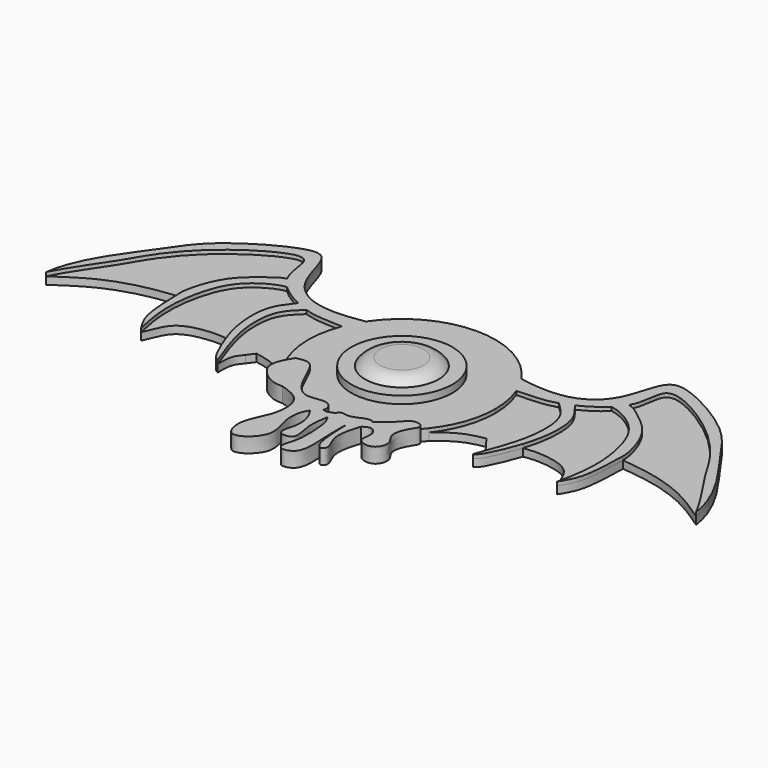
from build123d import *

# Parameters (mm, degrees)
F1_DEPTH  = 3
F2_R      = 13.5064277213
F3_DEPTH  = 5
F4_R      = 9.8042212389
F5_DEPTH  = 7
F7_DEPTH  = 2
F8_DEPTH  = 3
F10_DEPTH = 4


# Not quite as in the source:
# - a fillet or chamfer that OpenCascade refuses, or shapes differently, is made with other operations: its cross-section is extruded or revolved along the edge and cut away or added


with BuildPart() as f1:
    # F0 (on Top) → F1 (new body)
    with BuildSketch(Plane.XY):
        with BuildLine():
            ThreePointArc((-19.6218875172, -15.4913372651), (0, -25), (19.6218875172, -15.4913372651))
            add(Edge.make_bspline(
                [(20.7636337812, 13.92377507), (18.884492427, 12.8973675107), (13.2694896297, 9.830391573), (17.0839746859, -5.3747888898), (19.6218875172, -15.4913372651)],
                knots=[0, 0, 0, 0, 0.3346643665, 1, 1, 1, 1], degree=3))
            ThreePointArc((20.7636337812, 13.92377507), (0, 25), (-20.7636337812, 13.92377507))
            add(Edge.make_bspline(
                [(-20.7636337812, 13.92377507), (-18.884492427, 12.8973675107), (-13.2694896297, 9.830391573), (-17.0839746859, -5.3747888898), (-19.6218875172, -15.4913372651)],
                knots=[0, 0, 0, 0, 0.3346643665, 1, 1, 1, 1], degree=3))
        make_face()
        with BuildLine():
            ThreePointArc((19.6218875172, -15.4913372651), (23.61723087, -8.1991710578), (25, 0))
            ThreePointArc((25, 0), (24.5689951544, 4.6221723357), (23.2908418319, 9.0849703775))
            ThreePointArc((23.2908418319, 9.0849703775), (22.1597092287, 11.5735598197), (20.7636337812, 13.92377507))
            add(Edge.make_bspline(
                [(20.7636337812, 13.92377507), (18.884492427, 12.8973675107), (13.2694896297, 9.830391573), (17.0839746859, -5.3747888898), (19.6218875172, -15.4913372651)],
                knots=[0, 0, 0, 0, 0.3346643665, 1, 1, 1, 1], degree=3))
        make_face()
        with BuildLine():
            ThreePointArc((-23.2908418319, 9.0849703775), (-24.7259844978, -3.6912993126), (-19.6218875172, -15.4913372651))
            add(Edge.make_bspline(
                [(-20.7636337812, 13.92377507), (-18.884492427, 12.8973675107), (-13.2694896297, 9.830391573), (-17.0839746859, -5.3747888898), (-19.6218875172, -15.4913372651)],
                knots=[0, 0, 0, 0, 0.3346643665, 1, 1, 1, 1], degree=3))
            ThreePointArc((-20.7636337812, 13.92377507), (-22.1597092287, 11.5735598197), (-23.2908418319, 9.0849703775))
        make_face()
    extrude(amount=F1_DEPTH)

    # F2 (on Top) → F3 (join)
    with BuildSketch(Plane.XY):
        Circle(F2_R)
    extrude(amount=F3_DEPTH)

    # F4 (on Top) → F5 (join)
    with BuildSketch(Plane.XY):
        Circle(F4_R)
    extrude(amount=F5_DEPTH)

    # F6: fillet of radius 5 on 1 edges, made by hand

    # F6_s1 → F6_t2 (revolve, cut)
    with BuildSketch(Plane.XZ):
        with BuildLine():
            ThreePointArc((9.8042212389, 5), (8.0402892164, 6.472135955), (5.8042212389, 7))
            Line((5.8042212389, 7), (9.8042212389, 7))
            Line((9.8042212389, 7), (9.8042212389, 5))
        make_face()
    revolve(axis=Axis((0, 0, 7), (0, 0, 1)), mode=Mode.SUBTRACT)

    # F0 (on Top) → F7 (join)
    with BuildSketch(Plane.XY):
        with BuildLine():
            ThreePointArc((20.7636337812, 13.92377507), (22.1597092287, 11.5735598197), (23.2908418319, 9.0849703775))
            add(Edge.make_bspline(
                [(23.2908418319, 9.0849703775), (27.8215143515, 9.3257680742), (30.2320226011, 9.1590800923), (33.7177366018, 10.2821364999)],
                knots=[0, 0, 0, 0, 0.1231403921, 0.1231403921, 0.1231403921, 0.1231403921], degree=3))
            add(Edge.make_bspline(
                [(33.7177366018, 10.2821364999), (34.7454077104, 10.6132401484), (35.866536795, 11.0564496893), (37.004531993, 11.5978625395)],
                knots=[0.1231403921, 0.1231403921, 0.1231403921, 0.1231403921, 0.1594450984, 0.1594450984, 0.1594450984, 0.1594450984], degree=3))
            add(Edge.make_bspline(
                [(37.004531993, 11.5978625395), (39.2474500295, 12.6649537267), (41.555886116, 14.1135251746), (43.3434300018, 15.8371345407)],
                knots=[0.1594450984, 0.1594450984, 0.1594450984, 0.1594450984, 0.2309994255, 0.2309994255, 0.2309994255, 0.2309994255], degree=3))
            add(Edge.make_bspline(
                [(43.3434300018, 15.8371345407), (44.2810928585, 16.7412603051), (45.0754287668, 17.7210645793), (45.641798526, 18.7611840665)],
                knots=[0.2309994255, 0.2309994255, 0.2309994255, 0.2309994255, 0.2685335165, 0.2685335165, 0.2685335165, 0.2685335165], degree=3))
            add(Edge.make_bspline(
                [(45.641798526, 18.7611840665), (47.3352689159, 21.8711868955), (46.777744727, 27.7747473366), (51.8560066338, 29.065553317), (66.3600577374, 20.2512677808), (74.7298542288, 9.6960609054), (77.7930462557, 3.5527051654), (84.7415977894, -6.1442317778), (86.8003591895, -10.2821364999)],
                knots=[0.2685335165, 0.2685335165, 0.2685335165, 0.2685335165, 0.3807620926, 0.4500912377, 0.6051903106, 0.7450551623, 0.8470726585, 1, 1, 1, 1], degree=3))
            add(Edge.make_bspline(
                [(20.7636337812, 13.92377507), (25.353260156, 13.083604301), (34.3722799665, 12.4739559617), (43.1666874947, 19.3658325346), (44.7883389447, 31.8865702273), (51.6235191398, 32.3410311281), (68.757647719, 22.5890249267), (75.2339965242, 11.4273433149), (85.5971213344, -1.5157287213), (86.8003591895, -10.2821364999)],
                knots=[0, 0, 0, 0, 0.1438051462, 0.2702269745, 0.4006587664, 0.4888335416, 0.6586500337, 0.8053535671, 1, 1, 1, 1], degree=3))
        make_face()
        with BuildLine():
            ThreePointArc((19.6218875172, -15.4913372651), (23.61723087, -8.1991710578), (25, 0))
            ThreePointArc((25, 0), (24.5689951544, 4.6221723357), (23.2908418319, 9.0849703775))
            ThreePointArc((23.2908418319, 9.0849703775), (22.1597092287, 11.5735598197), (20.7636337812, 13.92377507))
            add(Edge.make_bspline(
                [(20.7636337812, 13.92377507), (18.884492427, 12.8973675107), (13.2694896297, 9.830391573), (17.0839746859, -5.3747888898), (19.6218875172, -15.4913372651)],
                knots=[0, 0, 0, 0, 0.3346643665, 1, 1, 1, 1], degree=3))
        make_face()
        with BuildLine():
            ThreePointArc((23.2908418319, 9.0849703775), (24.5689951544, 4.6221723357), (25, 0))
            ThreePointArc((25, 0), (23.61723087, -8.1991710578), (19.6218875172, -15.4913372651))
            add(Edge.make_bspline(
                [(19.6218875172, -15.4913372651), (21.4152102231, -14.0609489213), (24.8604058768, -11.2746200768), (28.7928801922, -10.5001506768), (30.6888949126, -10.1227229461)],
                knots=[0, 0, 0, 0, 0.5172233423, 1, 1, 1, 1], degree=3))
            add(Edge.make_bspline(
                [(32.1116161516, -12.0142660523), (31.6373757386, -11.3837516835), (31.1631353256, -10.7532373148), (30.6888949126, -10.1227229461)],
                knots=[0, 0, 0, 0, 2.3668694612, 2.3668694612, 2.3668694612, 2.3668694612], degree=3))
            add(Edge.make_bspline(
                [(32.1116161516, -12.0142660523), (32.776720922, -12.8822985255), (34.1447409362, -14.3321949992), (34.1047637318, -17.2769145921), (34.0780636316, -18.8904348761)],
                knots=[0, 0, 0, 0, 0.4499025437, 1, 1, 1, 1], degree=3))
            add(Edge.make_bspline(
                [(33.7177366018, 10.2821364999), (35.3645415529, 8.7757476619), (38.884943387, 5.4848056386), (38.8140830901, -4.1284440887), (37.0736184249, -10.5819579136), (35.282158389, -15.8523198225), (34.0780636316, -18.8904348761)],
                knots=[0, 0, 0, 0, 0.2318500383, 0.4998701646, 0.7334854658, 1, 1, 1, 1], degree=3))
            add(Edge.make_bspline(
                [(23.2908418319, 9.0849703775), (27.8215143515, 9.3257680742), (30.2320226011, 9.1590800923), (33.7177366018, 10.2821364999)],
                knots=[0, 0, 0, 0, 0.1231403921, 0.1231403921, 0.1231403921, 0.1231403921], degree=3))
        make_face()
        with BuildLine():
            add(Edge.make_bspline(
                [(33.7177366018, 10.2821364999), (34.7454077104, 10.6132401484), (35.866536795, 11.0564496893), (37.004531993, 11.5978625395)],
                knots=[0.1231403921, 0.1231403921, 0.1231403921, 0.1231403921, 0.1594450984, 0.1594450984, 0.1594450984, 0.1594450984], degree=3))
            add(Edge.make_bspline(
                [(33.7177366018, 10.2821364999), (35.3645415529, 8.7757476619), (38.884943387, 5.4848056386), (38.8140830901, -4.1284440887), (37.0736184249, -10.5819579136), (35.282158389, -15.8523198225), (34.0780636316, -18.8904348761)],
                knots=[0, 0, 0, 0, 0.2318500383, 0.4998701646, 0.7334854658, 1, 1, 1, 1], degree=3))
            add(Edge.make_bspline(
                [(39.3599004471, -8.7854920866), (38.7249404903, -10.7452749087), (37.0180617267, -14.9012626381), (35.2493275964, -18.5335928874), (34.0780636316, -18.8904348761)],
                knots=[0.6277129418, 0.6277129418, 0.6277129418, 0.6277129418, 0.792816444, 1, 1, 1, 1], degree=3))
            add(Edge.make_bspline(
                [(37.004531993, 11.5978625395), (38.0800679502, 10.0046793736), (41.3336069296, 6.7268291074), (41.1834657071, -2.2502985215), (39.8295408824, -7.3359624778), (39.3599004471, -8.7854920866)],
                knots=[0, 0, 0, 0, 0.2173363693, 0.5055961378, 0.6277129418, 0.6277129418, 0.6277129418, 0.6277129418], degree=3))
        make_face()
        with BuildLine():
            add(Edge.make_bspline(
                [(37.004531993, 11.5978625395), (39.2474500295, 12.6649537267), (41.555886116, 14.1135251746), (43.3434300018, 15.8371345407)],
                knots=[0.1594450984, 0.1594450984, 0.1594450984, 0.1594450984, 0.2309994255, 0.2309994255, 0.2309994255, 0.2309994255], degree=3))
            add(Edge.make_bspline(
                [(37.004531993, 11.5978625395), (38.0800679502, 10.0046793736), (41.3336069296, 6.7268291074), (41.1834657071, -2.2502985215), (39.8295408824, -7.3359624778), (39.3599004471, -8.7854920866)],
                knots=[0, 0, 0, 0, 0.2173363693, 0.5055961378, 0.6277129418, 0.6277129418, 0.6277129418, 0.6277129418], degree=3))
            add(Edge.make_bspline(
                [(55.5573105812, -17.6151320338), (54.4439075888, -14.9875635555), (52.9703835571, -10.411043477), (46.6717355198, -8.6507292972), (42.2245726074, -8.3797506367), (40.2332096515, -8.6600986878), (39.3599004471, -8.7854920866)],
                knots=[0, 0, 0, 0, 0.3047383368, 0.5764576192, 0.8133522424, 1, 1, 1, 1], degree=3))
            add(Edge.make_bspline(
                [(43.3434300018, 15.8371345407), (45.3565623966, 15.5676262825), (49.9854795603, 13.2408710445), (54.5376514308, 8.1613285539), (57.1013516863, -1.3778788699), (57.1238501467, -10.2186225385), (56.0702038202, -15.2273425566), (55.5573105812, -17.6151320338)],
                knots=[0, 0, 0, 0, 0.1860076727, 0.3714288806, 0.5926344587, 0.8055769314, 1, 1, 1, 1], degree=3))
        make_face()
        with BuildLine():
            add(Edge.make_bspline(
                [(45.641798526, 18.7611840665), (47.0236524725, 18.4958354205), (50.5733406235, 15.7663353525), (56.3104736797, 11.1079119823), (58.8622688049, 3.2726876511), (59.0809752339, 0.6245344364), (59.0938226065, 0)],
                knots=[0, 0, 0, 0, 0.146943127, 0.3231645985, 0.5131967694, 0.5724247553, 0.5724247553, 0.5724247553, 0.5724247553], degree=3))
            add(Edge.make_bspline(
                [(43.3434300018, 15.8371345407), (44.2810928585, 16.7412603051), (45.0754287668, 17.7210645793), (45.641798526, 18.7611840665)],
                knots=[0.2309994255, 0.2309994255, 0.2309994255, 0.2309994255, 0.2685335165, 0.2685335165, 0.2685335165, 0.2685335165], degree=3))
            add(Edge.make_bspline(
                [(43.3434300018, 15.8371345407), (45.3565623966, 15.5676262825), (49.9854795603, 13.2408710445), (54.5376514308, 8.1613285539), (57.1013516863, -1.3778788699), (57.1238501467, -10.2186225385), (56.0702038202, -15.2273425566), (55.5573105812, -17.6151320338)],
                knots=[0, 0, 0, 0, 0.1860076727, 0.3714288806, 0.5926344587, 0.8055769314, 1, 1, 1, 1], degree=3))
            add(Edge.make_bspline(
                [(59.0938226065, 0), (59.1104927586, -0.8103667818), (58.9358631638, -3.6588287886), (58.782367202, -12.4944121501), (56.5431938855, -16.0569735079), (55.5573105812, -17.6151320338)],
                knots=[0.5724247553, 0.5724247553, 0.5724247553, 0.5724247553, 0.6492762299, 0.8452276156, 1, 1, 1, 1], degree=3))
        make_face()
        with BuildLine():
            add(Edge.make_bspline(
                [(59.0938226065, 0), (62.0265888913, -0.341290779), (68.0943487487, -1.0474058551), (78.0033682979, -4.2880779786), (83.850491985, -8.272167765), (86.8003591895, -10.2821364999)],
                knots=[0, 0, 0, 0, 0.3167243267, 0.6552882052, 1, 1, 1, 1], degree=3))
            add(Edge.make_bspline(
                [(45.641798526, 18.7611840665), (47.3352689159, 21.8711868955), (46.777744727, 27.7747473366), (51.8560066338, 29.065553317), (66.3600577374, 20.2512677808), (74.7298542288, 9.6960609054), (77.7930462557, 3.5527051654), (84.7415977894, -6.1442317778), (86.8003591895, -10.2821364999)],
                knots=[0.2685335165, 0.2685335165, 0.2685335165, 0.2685335165, 0.3807620926, 0.4500912377, 0.6051903106, 0.7450551623, 0.8470726585, 1, 1, 1, 1], degree=3))
            add(Edge.make_bspline(
                [(45.641798526, 18.7611840665), (47.0236524725, 18.4958354205), (50.5733406235, 15.7663353525), (56.3104736797, 11.1079119823), (58.8622688049, 3.2726876511), (59.0809752339, 0.6245344364), (59.0938226065, 0)],
                knots=[0, 0, 0, 0, 0.146943127, 0.3231645985, 0.5131967694, 0.5724247553, 0.5724247553, 0.5724247553, 0.5724247553], degree=3))
        make_face()
        with BuildLine():
            add(Edge.make_bspline(
                [(-19.6218875172, -15.4913372651), (-21.4152102231, -14.0609489213), (-24.8604058768, -11.2746200768), (-28.7928801922, -10.5001506768), (-30.6888949126, -10.1227229461)],
                knots=[0, 0, 0, 0, 0.5172233423, 1, 1, 1, 1], degree=3))
            ThreePointArc((-19.6218875172, -15.4913372651), (-24.7259844978, -3.6912993126), (-23.2908418319, 9.0849703775))
            add(Edge.make_bspline(
                [(-23.2908418319, 9.0849703775), (-27.8215143515, 9.3257680742), (-30.2320226011, 9.1590800923), (-33.7177366018, 10.2821364999)],
                knots=[0, 0, 0, 0, 0.1231403921, 0.1231403921, 0.1231403921, 0.1231403921], degree=3))
            add(Edge.make_bspline(
                [(-33.7177366018, 10.2821364999), (-35.3645415529, 8.7757476619), (-38.884943387, 5.4848056386), (-38.8140830901, -4.1284440887), (-37.0736184249, -10.5819579136), (-35.282158389, -15.8523198225), (-34.0780636316, -18.8904348761)],
                knots=[0, 0, 0, 0, 0.2318500383, 0.4998701646, 0.7334854658, 1, 1, 1, 1], degree=3))
            add(Edge.make_bspline(
                [(-32.1116161516, -12.0142660523), (-32.776720922, -12.8822985255), (-34.1447409362, -14.3321949992), (-34.1047637318, -17.2769145921), (-34.0780636316, -18.8904348761)],
                knots=[0, 0, 0, 0, 0.4499025437, 1, 1, 1, 1], degree=3))
            add(Edge.make_bspline(
                [(-32.1116161516, -12.0142660523), (-31.6373757386, -11.3837516835), (-31.1631353256, -10.7532373148), (-30.6888949126, -10.1227229461)],
                knots=[0, 0, 0, 0, 2.3668694612, 2.3668694612, 2.3668694612, 2.3668694612], degree=3))
        make_face()
        with BuildLine():
            add(Edge.make_bspline(
                [(-37.004531993, 11.5978625395), (-38.0800679502, 10.0046793736), (-41.3336069296, 6.7268291074), (-41.1834657071, -2.2502985215), (-39.8295408824, -7.3359624778), (-39.3599004471, -8.7854920866)],
                knots=[0, 0, 0, 0, 0.2173363693, 0.5055961378, 0.6277129418, 0.6277129418, 0.6277129418, 0.6277129418], degree=3))
            add(Edge.make_bspline(
                [(-37.004531993, 11.5978625395), (-39.2474500295, 12.6649537267), (-41.555886116, 14.1135251746), (-43.3434300018, 15.8371345407)],
                knots=[0.1594450984, 0.1594450984, 0.1594450984, 0.1594450984, 0.2309994255, 0.2309994255, 0.2309994255, 0.2309994255], degree=3))
            add(Edge.make_bspline(
                [(-43.3434300018, 15.8371345407), (-45.3565623966, 15.5676262825), (-49.9854795603, 13.2408710445), (-54.5376514308, 8.1613285539), (-57.1013516863, -1.3778788699), (-57.1238501467, -10.2186225385), (-56.0702038202, -15.2273425566), (-55.5573105812, -17.6151320338)],
                knots=[0, 0, 0, 0, 0.1860076727, 0.3714288806, 0.5926344587, 0.8055769314, 1, 1, 1, 1], degree=3))
            add(Edge.make_bspline(
                [(-55.5573105812, -17.6151320338), (-54.4439075888, -14.9875635555), (-52.9703835571, -10.411043477), (-46.6717355198, -8.6507292972), (-42.2245726074, -8.3797506367), (-40.2332096515, -8.6600986878), (-39.3599004471, -8.7854920866)],
                knots=[0, 0, 0, 0, 0.3047383368, 0.5764576192, 0.8133522424, 1, 1, 1, 1], degree=3))
        make_face()
        with BuildLine():
            add(Edge.make_bspline(
                [(-33.7177366018, 10.2821364999), (-35.3645415529, 8.7757476619), (-38.884943387, 5.4848056386), (-38.8140830901, -4.1284440887), (-37.0736184249, -10.5819579136), (-35.282158389, -15.8523198225), (-34.0780636316, -18.8904348761)],
                knots=[0, 0, 0, 0, 0.2318500383, 0.4998701646, 0.7334854658, 1, 1, 1, 1], degree=3))
            add(Edge.make_bspline(
                [(-33.7177366018, 10.2821364999), (-34.7454077104, 10.6132401484), (-35.866536795, 11.0564496893), (-37.004531993, 11.5978625395)],
                knots=[0.1231403921, 0.1231403921, 0.1231403921, 0.1231403921, 0.1594450984, 0.1594450984, 0.1594450984, 0.1594450984], degree=3))
            add(Edge.make_bspline(
                [(-37.004531993, 11.5978625395), (-38.0800679502, 10.0046793736), (-41.3336069296, 6.7268291074), (-41.1834657071, -2.2502985215), (-39.8295408824, -7.3359624778), (-39.3599004471, -8.7854920866)],
                knots=[0, 0, 0, 0, 0.2173363693, 0.5055961378, 0.6277129418, 0.6277129418, 0.6277129418, 0.6277129418], degree=3))
            add(Edge.make_bspline(
                [(-39.3599004471, -8.7854920866), (-38.7249404903, -10.7452749087), (-37.0180617267, -14.9012626381), (-35.2493275964, -18.5335928874), (-34.0780636316, -18.8904348761)],
                knots=[0.6277129418, 0.6277129418, 0.6277129418, 0.6277129418, 0.792816444, 1, 1, 1, 1], degree=3))
        make_face()
        with BuildLine():
            ThreePointArc((-23.2908418319, 9.0849703775), (-22.1597092287, 11.5735598197), (-20.7636337812, 13.92377507))
            add(Edge.make_bspline(
                [(-20.7636337812, 13.92377507), (-25.353260156, 13.083604301), (-34.3722799665, 12.4739559617), (-43.1666874947, 19.3658325346), (-44.7883389447, 31.8865702273), (-51.6235191398, 32.3410311281), (-68.757647719, 22.5890249267), (-75.2339965242, 11.4273433149), (-85.5971213344, -1.5157287213), (-86.8003591895, -10.2821364999)],
                knots=[0, 0, 0, 0, 0.1438051462, 0.2702269745, 0.4006587664, 0.4888335416, 0.6586500337, 0.8053535671, 1, 1, 1, 1], degree=3))
            add(Edge.make_bspline(
                [(-45.641798526, 18.7611840665), (-47.3352689159, 21.8711868955), (-46.777744727, 27.7747473366), (-51.8560066338, 29.065553317), (-66.3600577374, 20.2512677808), (-74.7298542288, 9.6960609054), (-77.7930462557, 3.5527051654), (-84.7415977894, -6.1442317778), (-86.8003591895, -10.2821364999)],
                knots=[0.2685335165, 0.2685335165, 0.2685335165, 0.2685335165, 0.3807620926, 0.4500912377, 0.6051903106, 0.7450551623, 0.8470726585, 1, 1, 1, 1], degree=3))
            add(Edge.make_bspline(
                [(-43.3434300018, 15.8371345407), (-44.2810928585, 16.7412603051), (-45.0754287668, 17.7210645793), (-45.641798526, 18.7611840665)],
                knots=[0.2309994255, 0.2309994255, 0.2309994255, 0.2309994255, 0.2685335165, 0.2685335165, 0.2685335165, 0.2685335165], degree=3))
            add(Edge.make_bspline(
                [(-37.004531993, 11.5978625395), (-39.2474500295, 12.6649537267), (-41.555886116, 14.1135251746), (-43.3434300018, 15.8371345407)],
                knots=[0.1594450984, 0.1594450984, 0.1594450984, 0.1594450984, 0.2309994255, 0.2309994255, 0.2309994255, 0.2309994255], degree=3))
            add(Edge.make_bspline(
                [(-33.7177366018, 10.2821364999), (-34.7454077104, 10.6132401484), (-35.866536795, 11.0564496893), (-37.004531993, 11.5978625395)],
                knots=[0.1231403921, 0.1231403921, 0.1231403921, 0.1231403921, 0.1594450984, 0.1594450984, 0.1594450984, 0.1594450984], degree=3))
            add(Edge.make_bspline(
                [(-23.2908418319, 9.0849703775), (-27.8215143515, 9.3257680742), (-30.2320226011, 9.1590800923), (-33.7177366018, 10.2821364999)],
                knots=[0, 0, 0, 0, 0.1231403921, 0.1231403921, 0.1231403921, 0.1231403921], degree=3))
        make_face()
        with BuildLine():
            add(Edge.make_bspline(
                [(-45.641798526, 18.7611840665), (-47.3352689159, 21.8711868955), (-46.777744727, 27.7747473366), (-51.8560066338, 29.065553317), (-66.3600577374, 20.2512677808), (-74.7298542288, 9.6960609054), (-77.7930462557, 3.5527051654), (-84.7415977894, -6.1442317778), (-86.8003591895, -10.2821364999)],
                knots=[0.2685335165, 0.2685335165, 0.2685335165, 0.2685335165, 0.3807620926, 0.4500912377, 0.6051903106, 0.7450551623, 0.8470726585, 1, 1, 1, 1], degree=3))
            add(Edge.make_bspline(
                [(-59.0938226065, 0), (-62.0265888913, -0.341290779), (-68.0943487487, -1.0474058551), (-78.0033682979, -4.2880779786), (-83.850491985, -8.272167765), (-86.8003591895, -10.2821364999)],
                knots=[0, 0, 0, 0, 0.3167243267, 0.6552882052, 1, 1, 1, 1], degree=3))
            add(Edge.make_bspline(
                [(-45.641798526, 18.7611840665), (-47.0236524725, 18.4958354205), (-50.5733406235, 15.7663353525), (-56.3104736797, 11.1079119823), (-58.8622688049, 3.2726876511), (-59.0809752339, 0.6245344364), (-59.0938226065, 0)],
                knots=[0, 0, 0, 0, 0.146943127, 0.3231645985, 0.5131967694, 0.5724247553, 0.5724247553, 0.5724247553, 0.5724247553], degree=3))
        make_face()
        with BuildLine():
            add(Edge.make_bspline(
                [(-43.3434300018, 15.8371345407), (-44.2810928585, 16.7412603051), (-45.0754287668, 17.7210645793), (-45.641798526, 18.7611840665)],
                knots=[0.2309994255, 0.2309994255, 0.2309994255, 0.2309994255, 0.2685335165, 0.2685335165, 0.2685335165, 0.2685335165], degree=3))
            add(Edge.make_bspline(
                [(-45.641798526, 18.7611840665), (-47.0236524725, 18.4958354205), (-50.5733406235, 15.7663353525), (-56.3104736797, 11.1079119823), (-58.8622688049, 3.2726876511), (-59.0809752339, 0.6245344364), (-59.0938226065, 0)],
                knots=[0, 0, 0, 0, 0.146943127, 0.3231645985, 0.5131967694, 0.5724247553, 0.5724247553, 0.5724247553, 0.5724247553], degree=3))
            add(Edge.make_bspline(
                [(-59.0938226065, 0), (-59.1104927586, -0.8103667818), (-58.9358631638, -3.6588287886), (-58.782367202, -12.4944121501), (-56.5431938855, -16.0569735079), (-55.5573105812, -17.6151320338)],
                knots=[0.5724247553, 0.5724247553, 0.5724247553, 0.5724247553, 0.6492762299, 0.8452276156, 1, 1, 1, 1], degree=3))
            add(Edge.make_bspline(
                [(-43.3434300018, 15.8371345407), (-45.3565623966, 15.5676262825), (-49.9854795603, 13.2408710445), (-54.5376514308, 8.1613285539), (-57.1013516863, -1.3778788699), (-57.1238501467, -10.2186225385), (-56.0702038202, -15.2273425566), (-55.5573105812, -17.6151320338)],
                knots=[0, 0, 0, 0, 0.1860076727, 0.3714288806, 0.5926344587, 0.8055769314, 1, 1, 1, 1], degree=3))
        make_face()
        with BuildLine():
            ThreePointArc((-23.2908418319, 9.0849703775), (-24.7259844978, -3.6912993126), (-19.6218875172, -15.4913372651))
            add(Edge.make_bspline(
                [(-20.7636337812, 13.92377507), (-18.884492427, 12.8973675107), (-13.2694896297, 9.830391573), (-17.0839746859, -5.3747888898), (-19.6218875172, -15.4913372651)],
                knots=[0, 0, 0, 0, 0.3346643665, 1, 1, 1, 1], degree=3))
            ThreePointArc((-20.7636337812, 13.92377507), (-22.1597092287, 11.5735598197), (-23.2908418319, 9.0849703775))
        make_face()
    extrude(amount=F7_DEPTH)

    # F0 (on Top) → F8 (join)
    with BuildSketch(Plane.XY):
        with BuildLine():
            ThreePointArc((20.7636337812, 13.92377507), (22.1597092287, 11.5735598197), (23.2908418319, 9.0849703775))
            add(Edge.make_bspline(
                [(23.2908418319, 9.0849703775), (27.8215143515, 9.3257680742), (30.2320226011, 9.1590800923), (33.7177366018, 10.2821364999)],
                knots=[0, 0, 0, 0, 0.1231403921, 0.1231403921, 0.1231403921, 0.1231403921], degree=3))
            add(Edge.make_bspline(
                [(33.7177366018, 10.2821364999), (34.7454077104, 10.6132401484), (35.866536795, 11.0564496893), (37.004531993, 11.5978625395)],
                knots=[0.1231403921, 0.1231403921, 0.1231403921, 0.1231403921, 0.1594450984, 0.1594450984, 0.1594450984, 0.1594450984], degree=3))
            add(Edge.make_bspline(
                [(37.004531993, 11.5978625395), (39.2474500295, 12.6649537267), (41.555886116, 14.1135251746), (43.3434300018, 15.8371345407)],
                knots=[0.1594450984, 0.1594450984, 0.1594450984, 0.1594450984, 0.2309994255, 0.2309994255, 0.2309994255, 0.2309994255], degree=3))
            add(Edge.make_bspline(
                [(43.3434300018, 15.8371345407), (44.2810928585, 16.7412603051), (45.0754287668, 17.7210645793), (45.641798526, 18.7611840665)],
                knots=[0.2309994255, 0.2309994255, 0.2309994255, 0.2309994255, 0.2685335165, 0.2685335165, 0.2685335165, 0.2685335165], degree=3))
            add(Edge.make_bspline(
                [(45.641798526, 18.7611840665), (47.3352689159, 21.8711868955), (46.777744727, 27.7747473366), (51.8560066338, 29.065553317), (66.3600577374, 20.2512677808), (74.7298542288, 9.6960609054), (77.7930462557, 3.5527051654), (84.7415977894, -6.1442317778), (86.8003591895, -10.2821364999)],
                knots=[0.2685335165, 0.2685335165, 0.2685335165, 0.2685335165, 0.3807620926, 0.4500912377, 0.6051903106, 0.7450551623, 0.8470726585, 1, 1, 1, 1], degree=3))
            add(Edge.make_bspline(
                [(20.7636337812, 13.92377507), (25.353260156, 13.083604301), (34.3722799665, 12.4739559617), (43.1666874947, 19.3658325346), (44.7883389447, 31.8865702273), (51.6235191398, 32.3410311281), (68.757647719, 22.5890249267), (75.2339965242, 11.4273433149), (85.5971213344, -1.5157287213), (86.8003591895, -10.2821364999)],
                knots=[0, 0, 0, 0, 0.1438051462, 0.2702269745, 0.4006587664, 0.4888335416, 0.6586500337, 0.8053535671, 1, 1, 1, 1], degree=3))
        make_face()
        with BuildLine():
            add(Edge.make_bspline(
                [(33.7177366018, 10.2821364999), (34.7454077104, 10.6132401484), (35.866536795, 11.0564496893), (37.004531993, 11.5978625395)],
                knots=[0.1231403921, 0.1231403921, 0.1231403921, 0.1231403921, 0.1594450984, 0.1594450984, 0.1594450984, 0.1594450984], degree=3))
            add(Edge.make_bspline(
                [(33.7177366018, 10.2821364999), (35.3645415529, 8.7757476619), (38.884943387, 5.4848056386), (38.8140830901, -4.1284440887), (37.0736184249, -10.5819579136), (35.282158389, -15.8523198225), (34.0780636316, -18.8904348761)],
                knots=[0, 0, 0, 0, 0.2318500383, 0.4998701646, 0.7334854658, 1, 1, 1, 1], degree=3))
            add(Edge.make_bspline(
                [(39.3599004471, -8.7854920866), (38.7249404903, -10.7452749087), (37.0180617267, -14.9012626381), (35.2493275964, -18.5335928874), (34.0780636316, -18.8904348761)],
                knots=[0.6277129418, 0.6277129418, 0.6277129418, 0.6277129418, 0.792816444, 1, 1, 1, 1], degree=3))
            add(Edge.make_bspline(
                [(37.004531993, 11.5978625395), (38.0800679502, 10.0046793736), (41.3336069296, 6.7268291074), (41.1834657071, -2.2502985215), (39.8295408824, -7.3359624778), (39.3599004471, -8.7854920866)],
                knots=[0, 0, 0, 0, 0.2173363693, 0.5055961378, 0.6277129418, 0.6277129418, 0.6277129418, 0.6277129418], degree=3))
        make_face()
        with BuildLine():
            add(Edge.make_bspline(
                [(45.641798526, 18.7611840665), (47.0236524725, 18.4958354205), (50.5733406235, 15.7663353525), (56.3104736797, 11.1079119823), (58.8622688049, 3.2726876511), (59.0809752339, 0.6245344364), (59.0938226065, 0)],
                knots=[0, 0, 0, 0, 0.146943127, 0.3231645985, 0.5131967694, 0.5724247553, 0.5724247553, 0.5724247553, 0.5724247553], degree=3))
            add(Edge.make_bspline(
                [(43.3434300018, 15.8371345407), (44.2810928585, 16.7412603051), (45.0754287668, 17.7210645793), (45.641798526, 18.7611840665)],
                knots=[0.2309994255, 0.2309994255, 0.2309994255, 0.2309994255, 0.2685335165, 0.2685335165, 0.2685335165, 0.2685335165], degree=3))
            add(Edge.make_bspline(
                [(43.3434300018, 15.8371345407), (45.3565623966, 15.5676262825), (49.9854795603, 13.2408710445), (54.5376514308, 8.1613285539), (57.1013516863, -1.3778788699), (57.1238501467, -10.2186225385), (56.0702038202, -15.2273425566), (55.5573105812, -17.6151320338)],
                knots=[0, 0, 0, 0, 0.1860076727, 0.3714288806, 0.5926344587, 0.8055769314, 1, 1, 1, 1], degree=3))
            add(Edge.make_bspline(
                [(59.0938226065, 0), (59.1104927586, -0.8103667818), (58.9358631638, -3.6588287886), (58.782367202, -12.4944121501), (56.5431938855, -16.0569735079), (55.5573105812, -17.6151320338)],
                knots=[0.5724247553, 0.5724247553, 0.5724247553, 0.5724247553, 0.6492762299, 0.8452276156, 1, 1, 1, 1], degree=3))
        make_face()
        with BuildLine():
            ThreePointArc((-23.2908418319, 9.0849703775), (-22.1597092287, 11.5735598197), (-20.7636337812, 13.92377507))
            add(Edge.make_bspline(
                [(-20.7636337812, 13.92377507), (-25.353260156, 13.083604301), (-34.3722799665, 12.4739559617), (-43.1666874947, 19.3658325346), (-44.7883389447, 31.8865702273), (-51.6235191398, 32.3410311281), (-68.757647719, 22.5890249267), (-75.2339965242, 11.4273433149), (-85.5971213344, -1.5157287213), (-86.8003591895, -10.2821364999)],
                knots=[0, 0, 0, 0, 0.1438051462, 0.2702269745, 0.4006587664, 0.4888335416, 0.6586500337, 0.8053535671, 1, 1, 1, 1], degree=3))
            add(Edge.make_bspline(
                [(-45.641798526, 18.7611840665), (-47.3352689159, 21.8711868955), (-46.777744727, 27.7747473366), (-51.8560066338, 29.065553317), (-66.3600577374, 20.2512677808), (-74.7298542288, 9.6960609054), (-77.7930462557, 3.5527051654), (-84.7415977894, -6.1442317778), (-86.8003591895, -10.2821364999)],
                knots=[0.2685335165, 0.2685335165, 0.2685335165, 0.2685335165, 0.3807620926, 0.4500912377, 0.6051903106, 0.7450551623, 0.8470726585, 1, 1, 1, 1], degree=3))
            add(Edge.make_bspline(
                [(-43.3434300018, 15.8371345407), (-44.2810928585, 16.7412603051), (-45.0754287668, 17.7210645793), (-45.641798526, 18.7611840665)],
                knots=[0.2309994255, 0.2309994255, 0.2309994255, 0.2309994255, 0.2685335165, 0.2685335165, 0.2685335165, 0.2685335165], degree=3))
            add(Edge.make_bspline(
                [(-37.004531993, 11.5978625395), (-39.2474500295, 12.6649537267), (-41.555886116, 14.1135251746), (-43.3434300018, 15.8371345407)],
                knots=[0.1594450984, 0.1594450984, 0.1594450984, 0.1594450984, 0.2309994255, 0.2309994255, 0.2309994255, 0.2309994255], degree=3))
            add(Edge.make_bspline(
                [(-33.7177366018, 10.2821364999), (-34.7454077104, 10.6132401484), (-35.866536795, 11.0564496893), (-37.004531993, 11.5978625395)],
                knots=[0.1231403921, 0.1231403921, 0.1231403921, 0.1231403921, 0.1594450984, 0.1594450984, 0.1594450984, 0.1594450984], degree=3))
            add(Edge.make_bspline(
                [(-23.2908418319, 9.0849703775), (-27.8215143515, 9.3257680742), (-30.2320226011, 9.1590800923), (-33.7177366018, 10.2821364999)],
                knots=[0, 0, 0, 0, 0.1231403921, 0.1231403921, 0.1231403921, 0.1231403921], degree=3))
        make_face()
        with BuildLine():
            add(Edge.make_bspline(
                [(-33.7177366018, 10.2821364999), (-35.3645415529, 8.7757476619), (-38.884943387, 5.4848056386), (-38.8140830901, -4.1284440887), (-37.0736184249, -10.5819579136), (-35.282158389, -15.8523198225), (-34.0780636316, -18.8904348761)],
                knots=[0, 0, 0, 0, 0.2318500383, 0.4998701646, 0.7334854658, 1, 1, 1, 1], degree=3))
            add(Edge.make_bspline(
                [(-33.7177366018, 10.2821364999), (-34.7454077104, 10.6132401484), (-35.866536795, 11.0564496893), (-37.004531993, 11.5978625395)],
                knots=[0.1231403921, 0.1231403921, 0.1231403921, 0.1231403921, 0.1594450984, 0.1594450984, 0.1594450984, 0.1594450984], degree=3))
            add(Edge.make_bspline(
                [(-37.004531993, 11.5978625395), (-38.0800679502, 10.0046793736), (-41.3336069296, 6.7268291074), (-41.1834657071, -2.2502985215), (-39.8295408824, -7.3359624778), (-39.3599004471, -8.7854920866)],
                knots=[0, 0, 0, 0, 0.2173363693, 0.5055961378, 0.6277129418, 0.6277129418, 0.6277129418, 0.6277129418], degree=3))
            add(Edge.make_bspline(
                [(-39.3599004471, -8.7854920866), (-38.7249404903, -10.7452749087), (-37.0180617267, -14.9012626381), (-35.2493275964, -18.5335928874), (-34.0780636316, -18.8904348761)],
                knots=[0.6277129418, 0.6277129418, 0.6277129418, 0.6277129418, 0.792816444, 1, 1, 1, 1], degree=3))
        make_face()
        with BuildLine():
            add(Edge.make_bspline(
                [(-43.3434300018, 15.8371345407), (-44.2810928585, 16.7412603051), (-45.0754287668, 17.7210645793), (-45.641798526, 18.7611840665)],
                knots=[0.2309994255, 0.2309994255, 0.2309994255, 0.2309994255, 0.2685335165, 0.2685335165, 0.2685335165, 0.2685335165], degree=3))
            add(Edge.make_bspline(
                [(-45.641798526, 18.7611840665), (-47.0236524725, 18.4958354205), (-50.5733406235, 15.7663353525), (-56.3104736797, 11.1079119823), (-58.8622688049, 3.2726876511), (-59.0809752339, 0.6245344364), (-59.0938226065, 0)],
                knots=[0, 0, 0, 0, 0.146943127, 0.3231645985, 0.5131967694, 0.5724247553, 0.5724247553, 0.5724247553, 0.5724247553], degree=3))
            add(Edge.make_bspline(
                [(-59.0938226065, 0), (-59.1104927586, -0.8103667818), (-58.9358631638, -3.6588287886), (-58.782367202, -12.4944121501), (-56.5431938855, -16.0569735079), (-55.5573105812, -17.6151320338)],
                knots=[0.5724247553, 0.5724247553, 0.5724247553, 0.5724247553, 0.6492762299, 0.8452276156, 1, 1, 1, 1], degree=3))
            add(Edge.make_bspline(
                [(-43.3434300018, 15.8371345407), (-45.3565623966, 15.5676262825), (-49.9854795603, 13.2408710445), (-54.5376514308, 8.1613285539), (-57.1013516863, -1.3778788699), (-57.1238501467, -10.2186225385), (-56.0702038202, -15.2273425566), (-55.5573105812, -17.6151320338)],
                knots=[0, 0, 0, 0, 0.1860076727, 0.3714288806, 0.5926344587, 0.8055769314, 1, 1, 1, 1], degree=3))
        make_face()
    extrude(amount=F8_DEPTH)

    # F9 (on Top) → F10 (join)
    with BuildSketch(Plane.XY):
        with BuildLine():
            add(Edge.make_bspline(
                [(-20.7235760014, -9.6445070811), (-19.40634346, -9.3306596256), (-16.2692731337, -8.5832173173), (-13.8404857628, -15.9262885752), (-9.3698744561, -22.893109603), (-2.8654473112, -19.9783646263), (-1.1182007603, -23.203626034), (-1.5408760969, -24.1634941887), (-1.6355179467, -24.3131122859)],
                knots=[0, 0, 0, 0, 0.0606496106, 0.1444511325, 0.2309256106, 0.3057439584, 0.3606752212, 0.3715110564, 0.3715110564, 0.3715110564, 0.3715110564], degree=3))
            add(Edge.make_bspline(
                [(-20.7235760014, -9.6445070811), (-21.9943953935, -11.7440305486), (-24.535062388, -15.9411575973), (-18.4930641439, -21.2411641402), (-15.918737994, -21.2695682893), (-14.8254489317, -21.2816298766)],
                knots=[0, 0, 0, 0, 0.3654142522, 0.7305034079, 1, 1, 1, 1], degree=3))
            add(Edge.make_bspline(
                [(-3.5070139238, -26.2158849673), (-4.6131211591, -27.5997100414), (-5.6895321201, -32.5921856123), (-1.5713967275, -40.0141150071), (-10.1452453114, -47.029797053), (-12.5639090643, -38.7870466023), (-7.9861304572, -32.4938336445), (-8.0062270704, -23.5381526959), (-12.6120485953, -22.0140884211), (-14.8254489317, -21.2816298766)],
                knots=[0.4169646347, 0.4169646347, 0.4169646347, 0.4169646347, 0.4958206062, 0.5846771067, 0.6693456642, 0.7426699508, 0.8329154656, 0.9197046813, 1, 1, 1, 1], degree=3))
            add(Edge.make_bspline(
                [(-1.6355179467, -24.3131122859), (-2.0325164873, -24.9407222314), (-2.8694397361, -25.418230708), (-3.5070139238, -26.2158849673)],
                knots=[0.3715110564, 0.3715110564, 0.3715110564, 0.3715110564, 0.4169646347, 0.4169646347, 0.4169646347, 0.4169646347], degree=3))
        make_face()
        with BuildLine():
            add(Edge.make_bspline(
                [(1.1985873829, -23.951514107), (0.9671167555, -23.8260086665), (-0.0754281046, -24.5534155095), (-1.0911163539, -24.3982023049), (-1.6355179467, -24.3131122859)],
                knots=[0.8691013178, 0.8691013178, 0.8691013178, 0.8691013178, 0.9301825186, 1, 1, 1, 1], degree=3))
            add(Edge.make_bspline(
                [(-1.6355179467, -24.3131122859), (-2.0325164873, -24.9407222314), (-2.8694397361, -25.418230708), (-3.5070139238, -26.2158849673)],
                knots=[0.3715110564, 0.3715110564, 0.3715110564, 0.3715110564, 0.4169646347, 0.4169646347, 0.4169646347, 0.4169646347], degree=3))
            add(Edge.make_bspline(
                [(-3.5070139238, -26.2158849673), (-2.883400909, -27.2108060416), (-1.5772187189, -29.3053951505), (-1.4367162452, -33.6612041083), (-2.8086719328, -36.8433496475), (-1.5821949157, -38.5187493793), (2.1045932294, -38.0152983382), (0.657934516, -33.3111620091), (0.6247250909, -29.5615780061), (1.0406939075, -27.2379166479), (1.1982494233, -26.2158849673)],
                knots=[0, 0, 0, 0, 0.1031682262, 0.2164685226, 0.3149071194, 0.3837004952, 0.4707341613, 0.580301166, 0.6920239127, 0.7820958486, 0.7820958486, 0.7820958486, 0.7820958486], degree=3))
            add(Edge.make_bspline(
                [(1.1982494233, -26.2158849673), (1.2225125476, -26.0584948459), (1.3705220613, -25.073510707), (1.4757351702, -24.1017861113), (1.1985873829, -23.951514107)],
                knots=[0.7820958486, 0.7820958486, 0.7820958486, 0.7820958486, 0.7959666837, 0.8691013178, 0.8691013178, 0.8691013178, 0.8691013178], degree=3))
        make_face()
        with BuildLine():
            add(Edge.make_bspline(
                [(1.1985873829, -23.951514107), (1.4456187322, -23.5413655037), (2.0607348171, -22.5172449826), (4.569693506, -23.6127308263), (7.6831118026, -21.5738187686), (9.5325944539, -21.6347257364), (9.8100658506, -22.1171975136)],
                knots=[0, 0, 0, 0, 0.0635011481, 0.1450475396, 0.250308378, 0.3247515807, 0.3247515807, 0.3247515807, 0.3247515807], degree=3))
            add(Edge.make_bspline(
                [(1.1982494233, -26.2158849673), (1.2225125476, -26.0584948459), (1.3705220613, -25.073510707), (1.4757351702, -24.1017861113), (1.1985873829, -23.951514107)],
                knots=[0.7820958486, 0.7820958486, 0.7820958486, 0.7820958486, 0.7959666837, 0.8691013178, 0.8691013178, 0.8691013178, 0.8691013178], degree=3))
            add(Edge.make_bspline(
                [(1.1982494233, -26.2158849673), (1.4979284081, -26.7344342174), (2.3511783621, -28.1806505644), (2.8960916753, -32.7060242963), (2.8368634421, -38.6304914955), (1.4698684717, -41.4487670686), (2.0468797086, -43.7835940306), (5.4960568497, -43.0399207048), (6.7358237459, -39.9814740684), (6.4991708276, -34.6131617172), (6.2124354964, -28.3028086529), (6.4117750153, -26.496719569)],
                knots=[0, 0, 0, 0, 0.081756919, 0.2032537912, 0.342202672, 0.4415256683, 0.5150852099, 0.6082203638, 0.7051553265, 0.8401046214, 1, 1, 1, 1], degree=3))
            add(Edge.make_bspline(
                [(9.3381456619, -25.2787085652), (9.196995182, -25.7167954283), (8.3192847319, -28.3791876849), (7.4811663995, -32.8328210461), (10.1657650242, -36.4540025692), (9.0159326644, -38.4196952544), (6.5383496697, -36.8673925358), (6.477853092, -29.0292938872), (6.4117750153, -26.496719569)],
                knots=[0.4130127364, 0.4130127364, 0.4130127364, 0.4130127364, 0.4411392496, 0.5778350075, 0.6865397452, 0.751044758, 0.8255380089, 1, 1, 1, 1], degree=3))
            add(Edge.make_bspline(
                [(9.8100658506, -22.1171975136), (10.1390407634, -22.6892244421), (9.7810766576, -23.9039895378), (9.3381456619, -25.2787085652)],
                knots=[0.3247515807, 0.3247515807, 0.3247515807, 0.3247515807, 0.4130127364, 0.4130127364, 0.4130127364, 0.4130127364], degree=3))
        make_face()
        with BuildLine():
            add(Edge.make_bspline(
                [(9.8100658506, -22.1171975136), (10.9741769979, -21.366557591), (13.3243177082, -19.8511443672), (15.9380704568, -15.7619444396), (19.975953422, -17.2572525302), (17.132914924, -20.4315107657), (16.1901407251, -24.7358698707), (19.1658910663, -27.1540254755), (17.5214979585, -31.8211786857), (11.9489568899, -30.4732240064), (13.8499253148, -26.3691078042), (11.419900129, -23.9422267652), (10.0144666281, -24.8453806809), (9.3381456619, -25.2787085652)],
                knots=[0, 0, 0, 0, 0.1021114388, 0.2061563584, 0.2845912757, 0.3745199668, 0.4749543371, 0.5648277156, 0.6592223078, 0.7554885334, 0.8480624308, 0.9269925885, 1, 1, 1, 1], degree=3))
            add(Edge.make_bspline(
                [(9.8100658506, -22.1171975136), (10.1390407634, -22.6892244421), (9.7810766576, -23.9039895378), (9.3381456619, -25.2787085652)],
                knots=[0.3247515807, 0.3247515807, 0.3247515807, 0.3247515807, 0.4130127364, 0.4130127364, 0.4130127364, 0.4130127364], degree=3))
        make_face()
    extrude(amount=F10_DEPTH)


solid = f1.part
